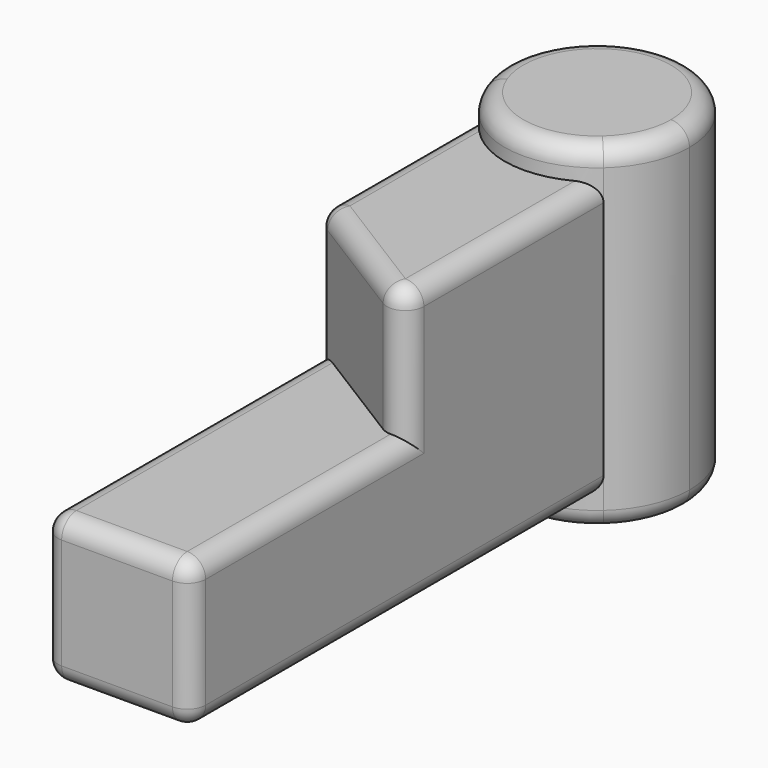
from build123d import *

# Parameters (mm, degrees)
F0_R     = 10
F1_DEPTH = 50
F2_DEPTH = 5
F3_DEPTH = 45
F4_DEPTH = 24
F5_DEPTH = 34.3
F6_R     = 3


with BuildPart() as f1:
    # F0 (on Top) → F1 (new body)
    with BuildSketch(Plane.XY):
        with BuildLine():
            ThreePointArc((10, 22.947157), (13.693064, 28.003773), (15, 34.127497))
            ThreePointArc((15, 34.127497), (-2.738613, 48.875378), (-14, 28.742332))
            ThreePointArc((-14, 28.742332), (-3.520797, 19.546551), (10, 22.947157))
        make_face()
        with Locations((0, 34.127497)):
            Circle(F0_R, mode=Mode.SUBTRACT)
        with Locations((0, 34.127497)):
            Circle(F0_R)
    extrude(amount=F1_DEPTH)

    # F0 (on Top) → F2 (join)
    with BuildSketch(Plane.XY):
        with BuildLine():
            ThreePointArc((10, 22.947157), (13.693064, 28.003773), (15, 34.127497))
            ThreePointArc((15, 34.127497), (-2.738613, 48.875378), (-14, 28.742332))
            ThreePointArc((-14, 28.742332), (-3.520797, 19.546551), (10, 22.947157))
        make_face()
        with Locations((0, 34.127497)):
            Circle(F0_R, mode=Mode.SUBTRACT)
        with Locations((0, 34.127497)):
            Circle(F0_R)
    extrude(amount=-F2_DEPTH)

    # F0 (on Top) → F3 (join)
    with BuildSketch(Plane.XY):
        with BuildLine():
            ThreePointArc((10, 22.947157), (-3.520797, 19.546551), (-14, 28.742332))
            Line((-14, 28.742332), (-14, -3.987999))
            Line((-14, -3.987999), (10, -18.962673))
            Line((10, -18.962673), (10, 22.947157))
        make_face()
    extrude(amount=F3_DEPTH)

    # F0 (on Top) → F4 (join)
    with BuildSketch(Plane.XY):
        Polygon((10, -18.962673), (-14, -3.987999), (-14, -60.872503), (10, -60.872503), align=None)
    extrude(amount=F4_DEPTH)

    # F0 (on Top) → F5 (cut, symmetric)
    with BuildSketch(Plane.XY):
        with Locations((0, 34.127497)):
            Circle(F0_R)
    extrude(amount=F5_DEPTH, both=True, mode=Mode.SUBTRACT)

    # F6
    f6_edges = [f1.edges().sort_by_distance(p)[0] for p in [
        (-14, 12.377166, 45),
        (-14, -3.987999, 34.5),
        (-2, -11.475336, 45),
        (10, 1.992242, 45),
        (-14, -32.430251, 24),
        (10, -39.917588, 24),
        (-2, -60.872503, 24),
        (10, -60.872503, 12),
        (-14, -60.872503, 12),
        (-2, -60.872503, 0),
        (-14, -16.065085, 0),
        (10, -18.962673, 34.5),
        (10, -18.962673, 0),
        (-15, 34.127497, -5),
        (-15, 34.127497, 50),
    ]]
    fillet(f6_edges, radius=F6_R)


solid = f1.part
